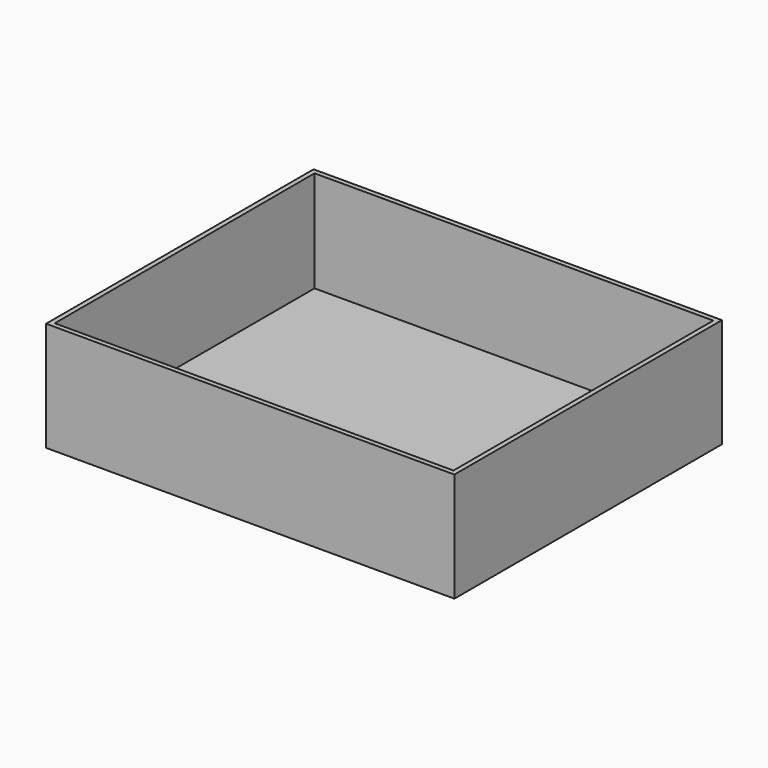
from build123d import *

# Parameters (mm, degrees)
F0_W     = 806.45
F0_H     = 215.9
F1_DEPTH = 660.4
F2_W     = 781.05
F2_H     = 641.35
F3_DEPTH = 6.35
F4_T     = -9.525


# Not quite as in the source:
# - a shell that OpenCascade refuses in one call is made with other operations: the cavity is built on its own and cut out


with BuildPart() as f1:
    # F0 (on Front) → F1 (new body)
    with BuildSketch(Plane.XZ):
        Rectangle(F0_W, F0_H)
    extrude(amount=F1_DEPTH)

    # F2 (on face) → F3 (cut)
    with BuildSketch(Plane(origin=(0, 0, -107.95), x_dir=(1, 0, 0), z_dir=(0, 0, -1))):
        with Locations((0, 330.2)):
            Rectangle(F2_W, F2_H)
    extrude(amount=-F3_DEPTH, mode=Mode.SUBTRACT)

    # F4: a shell. OpenCascade refuses it in one call, so the cavity is built on its own and cut out:
    # the body offset inwards by the wall thickness, plus a prism from it out through each open face.
    f4_core = offset(f1.part, amount=F4_T, kind=Kind.INTERSECTION, mode=Mode.PRIVATE)
    f4_exits = [f4_core.faces().sort_by_distance(p)[0] for p in [
        (0, -330.2, 98.425),
    ]]
    add(f4_core, mode=Mode.SUBTRACT)
    extrude(f4_exits, amount=-F4_T, mode=Mode.SUBTRACT)


solid = f1.part
